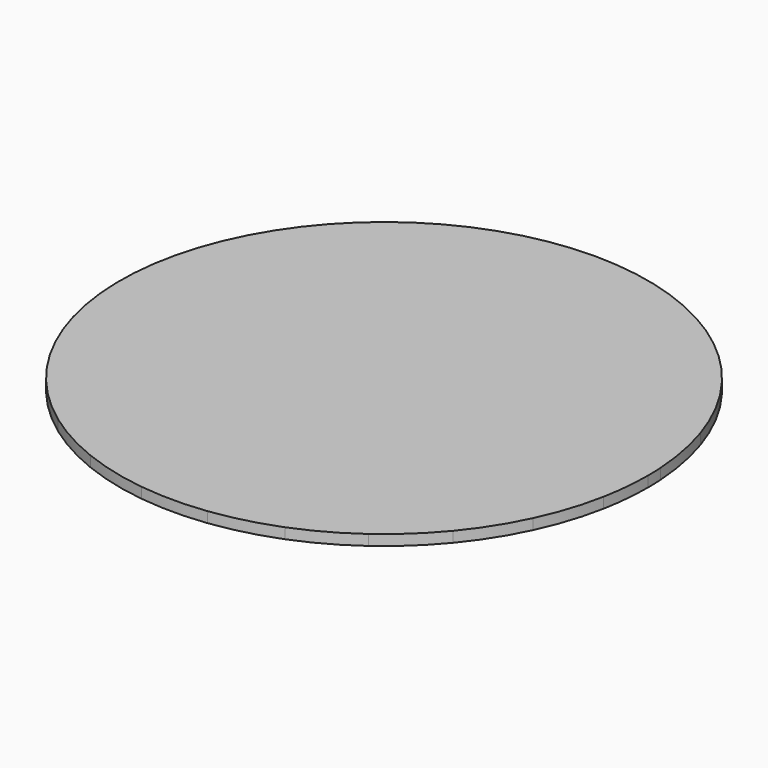
from build123d import *

# Parameters (mm, degrees)
F1_DEPTH = 0.26


with BuildPart() as f1:
    # F0 (on Top) → F1 (new body)
    with BuildSketch(Plane.XY):
        with BuildLine():
            ThreePointArc((6.5, 0), (6.4967926424, 0.204169934), (6.4871737348, 0.4081383769))
            ThreePointArc((6.4871737348, 0.4081383769), (6.3848671297, 1.2179785448), (6.1818673559, 2.0086104634))
            ThreePointArc((6.1818673559, 2.0086104634), (5.881375841, 2.7675653952), (5.4881315158, 3.4828741674))
            ThreePointArc((5.4881315158, 3.4828741674), (5.008336078, 4.1432559334), (4.4495561885, 4.7382960782))
            ThreePointArc((4.4495561885, 4.7382960782), (3.8206041399, 5.2586104634), (3.1313988817, 5.6959934203))
            ThreePointArc((3.1313988817, 5.6959934203), (2.3928095925, 6.0435471583), (1.6164842666, 6.2957905473))
            ThreePointArc((1.6164842666, 6.2957905473), (0.8146660182, 6.4487455585), (0, 6.5))
            ThreePointArc((0, 6.5), (-0.8146660182, 6.4487455585), (-1.6164842666, 6.2957905473))
            ThreePointArc((-1.6164842666, 6.2957905473), (-2.3928095925, 6.0435471583), (-3.1313988817, 5.6959934203))
            ThreePointArc((-3.1313988817, 5.6959934203), (-3.8206041399, 5.2586104634), (-4.4495561885, 4.7382960782))
            ThreePointArc((-4.4495561885, 4.7382960782), (-5.008336078, 4.1432559334), (-5.4881315158, 3.4828741674))
            ThreePointArc((-5.4881315158, 3.4828741674), (-5.881375841, 2.7675653952), (-6.1818673559, 2.0086104634))
            ThreePointArc((-6.1818673559, 2.0086104634), (-6.3848671297, 1.2179785448), (-6.4871737348, 0.4081383769))
            ThreePointArc((-6.4871737348, 0.4081383769), (-6.4871737348, -0.4081383769), (-6.3848671297, -1.2179785448))
            ThreePointArc((-6.3848671297, -1.2179785448), (-6.1818673559, -2.0086104634), (-5.881375841, -2.7675653952))
            ThreePointArc((-5.881375841, -2.7675653952), (-5.4881315158, -3.4828741674), (-5.008336078, -4.1432559334))
            ThreePointArc((-5.008336078, -4.1432559334), (-4.4495561885, -4.7382960782), (-3.8206041399, -5.2586104634))
            ThreePointArc((-3.8206041399, -5.2586104634), (-3.1313988817, -5.6959934203), (-2.3928095925, -6.0435471583))
            ThreePointArc((-2.3928095925, -6.0435471583), (-1.6164842666, -6.2957905473), (-0.8146660182, -6.4487455585))
            ThreePointArc((-0.8146660182, -6.4487455585), (0, -6.5), (0.8146660182, -6.4487455585))
            ThreePointArc((0.8146660182, -6.4487455585), (1.6164842666, -6.2957905473), (2.3928095925, -6.0435471583))
            ThreePointArc((2.3928095925, -6.0435471583), (3.1313988817, -5.6959934203), (3.8206041399, -5.2586104634))
            ThreePointArc((3.8206041399, -5.2586104634), (4.4495561885, -4.7382960782), (5.008336078, -4.1432559334))
            ThreePointArc((5.008336078, -4.1432559334), (5.4881315158, -3.4828741674), (5.881375841, -2.7675653952))
            ThreePointArc((5.881375841, -2.7675653952), (6.1818673559, -2.0086104634), (6.3848671297, -1.2179785448))
            ThreePointArc((6.3848671297, -1.2179785448), (6.4711527699, -0.6117040366), (6.5, 0))
        make_face()
    extrude(amount=F1_DEPTH)


solid = f1.part
